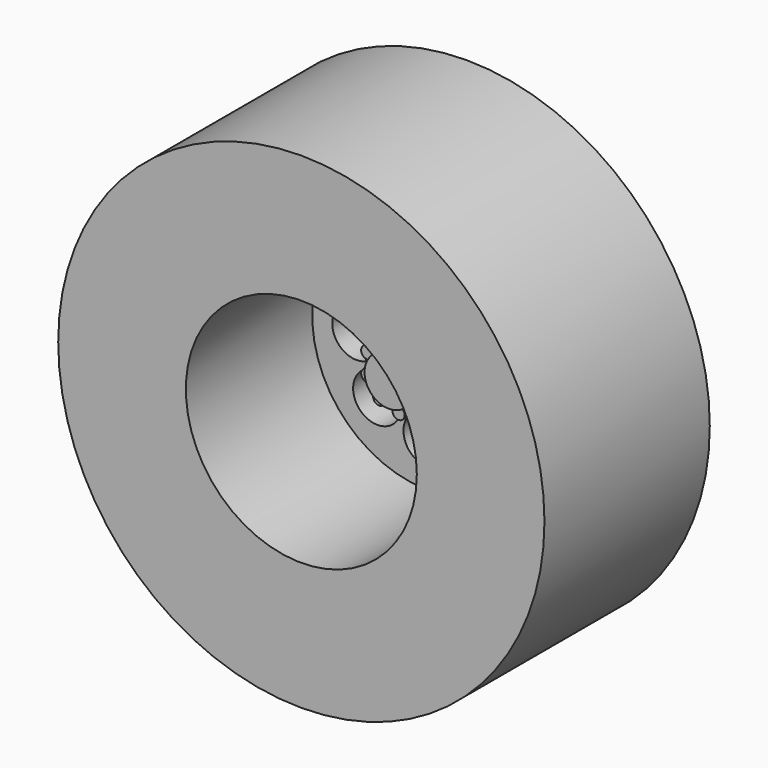
from build123d import *

# Parameters (mm, degrees)
F0_R      = 20
F1_DEPTH  = 17
F2_R      = 9.5
F3_DEPTH  = 13
F4_R      = 2
F5_DEPTH  = 4
F6_R      = 3.5
F7_DEPTH  = 2
F8_R      = 2
F9_DEPTH  = 2
F10_R     = 0.5
F11_DEPTH = 1
F12_R     = 3.5
F13_DEPTH = 9
F14_R     = 2.75
F15_DEPTH = 9
F16_R     = 19
F16_R_2   = 9.5
F17_DEPTH = 16
F18_R     = 10.25
F18_R_2   = 9.5
F19_DEPTH = 17


# Not quite as in the source:
# - a feature names something its author has since deleted; it is built from what else it names


with BuildPart() as f1:
    # F0 (on Front) → F1 (new body)
    with BuildSketch(Plane.XZ):
        Circle(F0_R)
    extrude(amount=F1_DEPTH)

    # F2 (on face) → F3 (cut)
    with BuildSketch(Plane.XZ.offset(17)):
        Circle(F2_R)
    extrude(amount=-F3_DEPTH, mode=Mode.SUBTRACT)

    # F4 (on face) → F5 (cut)
    with BuildSketch(Plane.XZ.offset(4)):
        with Locations((-4.1401582032, 4.1401582032)):
            Circle(F4_R)
        with Locations((0, 5.8550678814)):
            Circle(F4_R)
        with Locations((4.1401582032, 4.1401582032)):
            Circle(F4_R)
        with Locations((5.8550678814, 0)):
            Circle(F4_R)
        with Locations((4.1401582032, -4.1401582032)):
            Circle(F4_R)
        with Locations((0, -5.8550678814)):
            Circle(F4_R)
        with Locations((-4.1401582032, -4.1401582032)):
            Circle(F4_R)
        with Locations((-5.8550678814, 0)):
            Circle(F4_R)
    extrude(amount=-F5_DEPTH, mode=Mode.SUBTRACT)

    # F6 (on face) → F7 (join)
    with BuildSketch(Plane.XZ.offset(4)):
        Circle(F6_R)
    extrude(amount=F7_DEPTH)

    # F8 (on face) → F9 (join)
    with BuildSketch(Plane.XZ.offset(6)):
        Circle(F8_R)
    extrude(amount=F9_DEPTH)

    # F10 (on face) → F11 (join)
    with BuildSketch(Plane.XZ.offset(6)):
        with Locations((0, 2.7124709893)):
            Circle(F10_R)
        with Locations((1.5943504448, 2.1944351271)):
            Circle(F10_R)
        with Locations((2.5797132096, 0.8381996324)):
            Circle(F10_R)
        with Locations((2.5797132096, -0.8381996324)):
            Circle(F10_R)
        with Locations((1.5943504448, -2.1944351271)):
            Circle(F10_R)
        with Locations((0, -2.7124709893)):
            Circle(F10_R)
        with Locations((-1.5943504448, -2.1944351271)):
            Circle(F10_R)
        with Locations((-2.5797132096, -0.8381996324)):
            Circle(F10_R)
        with Locations((-2.5797132096, 0.8381996324)):
            Circle(F10_R)
        with Locations((-1.5943504448, 2.1944351271)):
            Circle(F10_R)
    extrude(amount=F11_DEPTH)

    # F12 (on face) → F13 (join)
    with BuildSketch(Plane(origin=(0, 0, 0), x_dir=(-1, 0, 0), z_dir=(0, 1, 0))):
        Circle(F12_R)
    extrude(amount=F13_DEPTH)

    # F14 (on face) → F15 (cut)
    with BuildSketch(Plane(origin=(0, 9, 0), x_dir=(-1, 0, 0), z_dir=(0, 1, 0))):
        Circle(F14_R)
    extrude(amount=-F15_DEPTH, mode=Mode.SUBTRACT)

    # F16 (on face) → F17 (cut)
    with BuildSketch(Plane(origin=(0, 0, 0), x_dir=(-1, 0, 0), z_dir=(0, 1, 0))):
        Circle(F16_R)
        Circle(F16_R_2, mode=Mode.SUBTRACT)
    extrude(amount=-F17_DEPTH, mode=Mode.SUBTRACT)

    # F18 (on face) → F19 (join)
    with BuildSketch(Plane.XZ.offset(17)):
        Circle(F18_R)
        Circle(F18_R_2, mode=Mode.SUBTRACT)
    extrude(amount=-F19_DEPTH)


solid = f1.part
